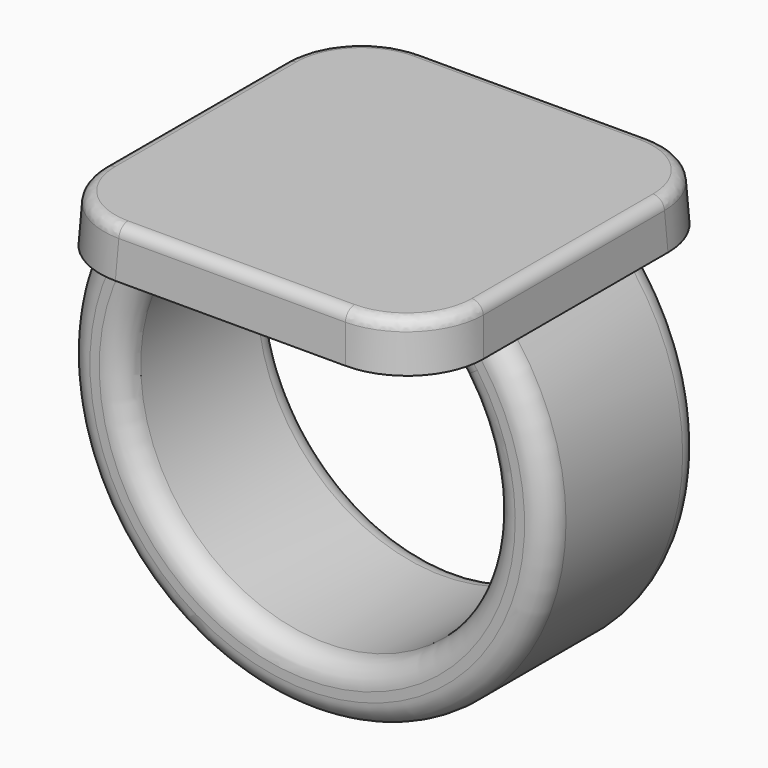
from build123d import *

# Parameters (mm, degrees)
F0_W     = 25.4
F0_H     = 25.4
F1_DEPTH = 3.175
F1_TAPER = 3
F3_W     = 5.08
F3_H     = 6.35
F6_DEPTH = 12.7
F7_R     = 5.08
F8_R     = 1.524
F9_R     = 0.762


with BuildPart() as f1:
    # F0 (on Top) → F1 (new body)
    with BuildSketch(Plane.XY):
        Rectangle(F0_W, F0_H)
    extrude(amount=F1_DEPTH, taper=F1_TAPER)

    # F4: sweep along a path in F2
    with BuildLine(Plane.XZ) as f4_path:
        ThreePointArc((-10.16, 0), (0, -23.5582897328), (10.16, 0))
    # F3 (on Top) → F4 (sweep)
    with BuildSketch(Plane.XY):
        with Locations((-10.16, -3.175)):
            Rectangle(F3_W, F3_H)
        with Locations((-10.16, 3.175)):
            Rectangle(F3_W, F3_H)
    sweep(path=f4_path.line)

    # F5 (on face) → F6 (join, through all)
    with BuildSketch(Plane.XZ.offset(6.35)):
        with BuildLine():
            ThreePointArc((10.0130578512, -2.535746045), (-1.743325406, -21.7110170055), (-7.62, 0))
            Line((-7.62, 0), (-12.7, 0))
            ThreePointArc((-12.7, 0), (0, -25.5013441222), (12.7, 0))
            Line((12.7, 0), (10.16, 0))
            Line((10.16, 0), (10.0130578512, -2.535746045))
        make_face()
        with BuildLine():
            ThreePointArc((7.62, 0), (8.9072265211, -1.1822790439), (10.0130578512, -2.535746045))
            Line((10.0130578512, -2.535746045), (10.16, 0))
            Line((10.16, 0), (7.62, 0))
        make_face()
    extrude(amount=-F6_DEPTH)

    # F7
    f7_edges = [f1.edges().sort_by_distance(p)[0] for p in [
        (12.616803, 12.616803, 1.5875),
        (-12.616803, 12.616803, 1.5875),
        (12.616803, -12.616803, 1.5875),
        (-12.616803, -12.616803, 1.5875),
    ]]
    fillet(f7_edges, radius=F7_R)

    # F8
    f8_edges = [f1.edges().sort_by_distance(p)[0] for p in [
        (0, -6.35, -21.835726),
        (0, -6.35, -25.501344),
        (0, 6.35, -25.501344),
        (0, 6.35, -21.835726),
    ]]
    fillet(f8_edges, radius=F8_R)

    # F9
    f9_edges = [f1.edges().sort_by_distance(p)[0] for p in [
        (0, 12.533605, 3.175),
        (11.048589, 11.048589, 3.175),
        (-11.048589, 11.048589, 3.175),
        (12.533605, 0, 3.175),
        (-12.533605, 0, 3.175),
        (11.048589, -11.048589, 3.175),
        (-11.048589, -11.048589, 3.175),
        (0, -12.533605, 3.175),
    ]]
    fillet(f9_edges, radius=F9_R)


solid = f1.part
